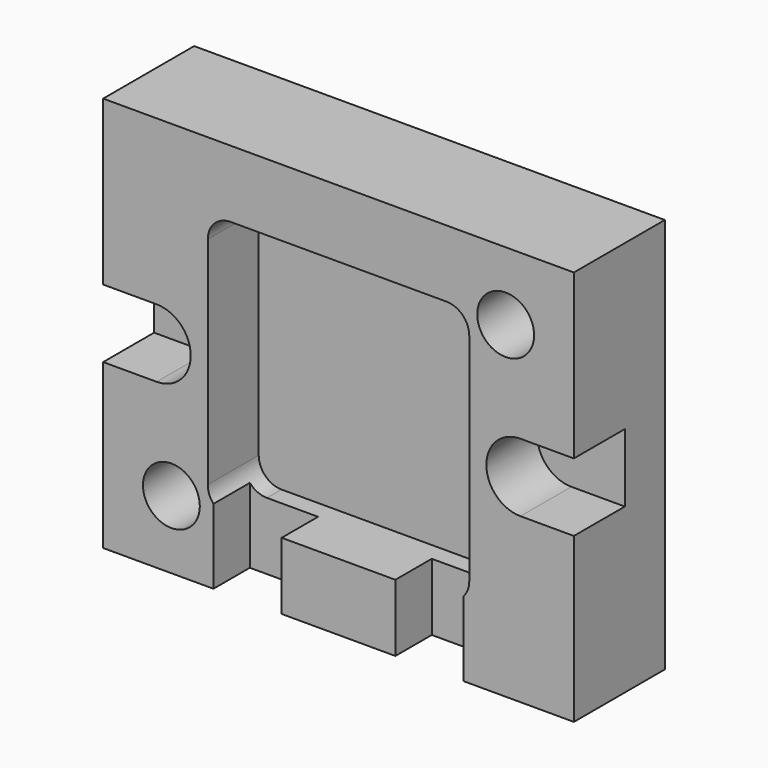
from build123d import *

# Parameters (mm, degrees)
F0_W           = 20.7
F0_H           = 17.4
F1_DEPTH       = 5
F2_W           = 11.5
F2_H           = 11.5
F3_DEPTH       = 2.8
F5_R           = 1
F7_DEPTH       = 2.8
F9_D           = 2.5
F9_DEPTH       = 5
F9_CBORE_D     = 4
F9_CBORE_DEPTH = 1.8
F9_TIP         = 0.7510757738
F11_DEPTH      = 2


# Not quite as in the source:
# - a feature names something its author has since deleted; it is built from what else it names


with BuildPart() as f1:
    # F0 (on Front) → F1 (new body)
    with BuildSketch(Plane.XZ):
        Rectangle(F0_W, F0_H)
    extrude(amount=-F1_DEPTH)

    # F2 (on face) → F3 (cut)
    with BuildSketch(Plane.XZ):
        Rectangle(F2_W, F2_H)
    extrude(amount=-F3_DEPTH, mode=Mode.SUBTRACT)

    # F5
    f5_edges = [f1.edges().sort_by_distance(p)[0] for p in [
        (-5.75, 1.4, 5.75),
        (5.75, 1.4, 5.75),
        (-5.75, 1.4, -5.75),
        (5.75, 1.4, -5.75),
    ]]
    fillet(f5_edges, radius=F5_R)

    # F6 (on face) → F7 (cut)
    with BuildSketch(Plane.XZ):
        with BuildLine():
            Line((-10.35, -1.5), (-8, -1.5))
            ThreePointArc((-8, -1.5), (-6.5, 0), (-8, 1.5))
            Line((-8, 1.5), (-10.35, 1.5))
            Line((-10.35, 1.5), (-10.35, -1.5))
        make_face()
        with BuildLine():
            ThreePointArc((8, 1.5), (6.5, 0), (8, -1.5))
            Line((8, -1.5), (8, 0))
            Line((8, 0), (8, 1.5))
        make_face()
        Polygon((8, -1.5), (10.35, -1.5), (10.35, 1.5), (8, 1.5), (8, 0), align=None)
    extrude(amount=-F7_DEPTH, mode=Mode.SUBTRACT)

    # F9
    with Locations(Plane(origin=(0, 5, 0), x_dir=(-1, 0, 0), z_dir=(0, 1, 0))):
        with Locations((7.35, -5.7), (-7.35, 5.7)):
            CounterBoreHole(F9_D / 2, F9_CBORE_D / 2, F9_CBORE_DEPTH, depth=F9_DEPTH)
            with Locations((0, 0, -(F9_DEPTH + F9_TIP / 2))):  # 118° drill point
                Cone(0, F9_D / 2, F9_TIP, mode=Mode.SUBTRACT)

    # F10 (on face) → F11 (cut)
    with BuildSketch(Plane.XZ):
        with BuildLine():
            Line((4.75, -5.75), (2.5, -5.75))
            Line((2.5, -5.75), (2.5, -8.7))
            Line((2.5, -8.7), (5.5, -8.7))
            Line((5.5, -8.7), (5.5, -5.4114378278))
            ThreePointArc((5.5, -5.4114378278), (5.1614378278, -5.6614378278), (4.75, -5.75))
        make_face()
        with BuildLine():
            Line((-2.5, -5.75), (-4.75, -5.75))
            ThreePointArc((-4.75, -5.75), (-5.1614378278, -5.6614378278), (-5.5, -5.4114378278))
            Line((-5.5, -5.4114378278), (-5.5, -8.7))
            Line((-5.5, -8.7), (-2.5, -8.7))
            Line((-2.5, -8.7), (-2.5, -5.75))
        make_face()
    extrude(amount=-F11_DEPTH, mode=Mode.SUBTRACT)


solid = f1.part
